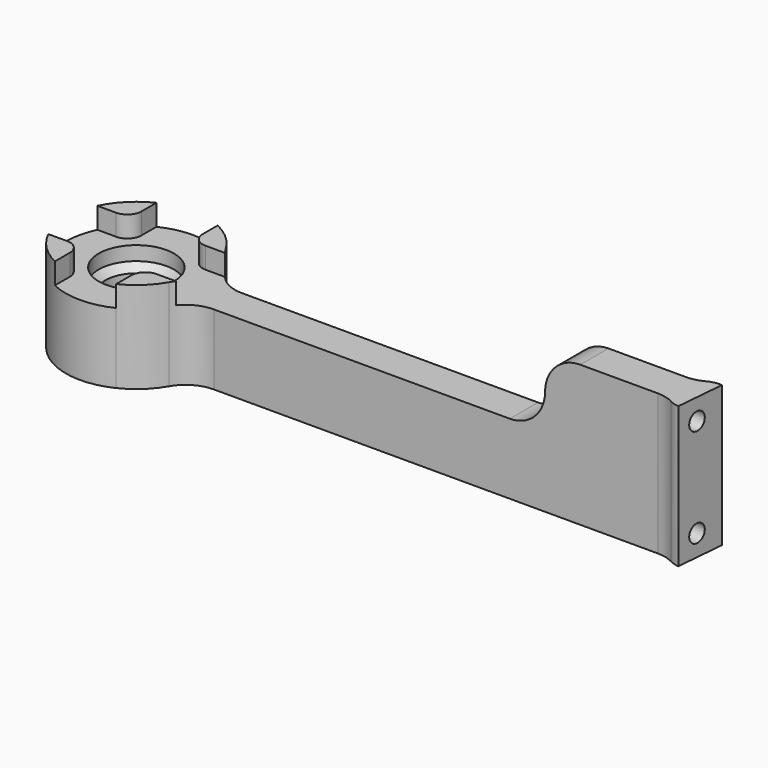
from build123d import *

# Parameters (mm, degrees)
F0_R         = 5.35
F1_DEPTH     = 10
F2_START     = 3.5
F0_R_2       = 4.35
F2_DEPTH     = 4.5
F3_SIZE      = 0.99999
F4_DEPTH     = 13
F5_DEPTH     = 20
F6_R         = 1.25
F7_DEPTH     = 7.5
F8_T1_DEPTH  = 20
F8_T3_DEPTH  = 5
F8_T8_DEPTH  = 10
F8_T13_DEPTH = 10
F8_T18_DEPTH = 18.2698067281
F8_T25_DEPTH = 10
F8_T30_DEPTH = 10
F8_T35_DEPTH = 18.2698067281
F8_T39_DEPTH = 30


# Not quite as in the source:
# - a fillet or chamfer that OpenCascade refuses, or shapes differently, is made with other operations: its cross-section is extruded or revolved along the edge and cut away or added
# - a fillet or chamfer is up to 0.001 mm smaller than in the source, because OpenCascade refuses the exact size


with BuildPart() as f1:
    # F0 (on Top) → F1 (new body)
    with BuildSketch(Plane.XY):
        with BuildLine():
            Line((-4.35, 6.35), (-4.35, 9.0043045262))
            ThreePointArc((-4.35, 9.0043045262), (-7.0710678119, 7.0710678119), (-9.0043045262, 4.35))
            Line((-9.0043045262, 4.35), (-6.35, 4.35))
            ThreePointArc((-6.35, 4.35), (-4.9357864376, 4.9357864376), (-4.35, 6.35))
        make_face()
        with BuildLine():
            ThreePointArc((9.6824583655, -2.5), (9.9202969627, -1.2600429248), (10, 0))
            ThreePointArc((10, 0), (9.9202969627, 1.2600429248), (9.6824583655, 2.5))
            ThreePointArc((9.6824583655, 2.5), (9.3890575588, 3.4417434764), (9.0043045262, 4.35))
            Line((9.0043045262, 4.35), (6.35, 4.35))
            ThreePointArc((6.35, 4.35), (4.9357864376, 4.9357864376), (4.35, 6.35))
            Line((4.35, 6.35), (4.35, 9.0043045262))
            ThreePointArc((4.35, 9.0043045262), (0, 10), (-4.35, 9.0043045262))
            Line((-4.35, 9.0043045262), (-4.35, 6.35))
            ThreePointArc((-4.35, 6.35), (-4.9357864376, 4.9357864376), (-6.35, 4.35))
            Line((-6.35, 4.35), (-9.0043045262, 4.35))
            ThreePointArc((-9.0043045262, 4.35), (-10, 0), (-9.0043045262, -4.35))
            Line((-9.0043045262, -4.35), (-6.35, -4.35))
            ThreePointArc((-6.35, -4.35), (-4.9357864376, -4.9357864376), (-4.35, -6.35))
            Line((-4.35, -6.35), (-4.35, -9.0043045262))
            ThreePointArc((-4.35, -9.0043045262), (0, -10), (4.35, -9.0043045262))
            Line((4.35, -9.0043045262), (4.35, -6.35))
            ThreePointArc((4.35, -6.35), (4.9357864376, -4.9357864376), (6.35, -4.35))
            Line((6.35, -4.35), (9.0043045262, -4.35))
            ThreePointArc((9.0043045262, -4.35), (9.3890575588, -3.4417434764), (9.6824583655, -2.5))
        make_face()
        Circle(F0_R, mode=Mode.SUBTRACT)
        with BuildLine():
            ThreePointArc((-9.0043045262, -4.35), (-7.0710678119, -7.0710678119), (-4.35, -9.0043045262))
            Line((-4.35, -9.0043045262), (-4.35, -6.35))
            ThreePointArc((-4.35, -6.35), (-4.9357864376, -4.9357864376), (-6.35, -4.35))
            Line((-6.35, -4.35), (-9.0043045262, -4.35))
        make_face()
        with BuildLine():
            ThreePointArc((4.35, -9.0043045262), (7.0710678119, -7.0710678119), (9.0043045262, -4.35))
            Line((9.0043045262, -4.35), (6.35, -4.35))
            ThreePointArc((6.35, -4.35), (4.9357864376, -4.9357864376), (4.35, -6.35))
            Line((4.35, -6.35), (4.35, -9.0043045262))
        make_face()
        with BuildLine():
            Line((6.35, 4.35), (9.0043045262, 4.35))
            ThreePointArc((9.0043045262, 4.35), (7.0710678119, 7.0710678119), (4.35, 9.0043045262))
            Line((4.35, 9.0043045262), (4.35, 6.35))
            ThreePointArc((4.35, 6.35), (4.9357864376, 4.9357864376), (6.35, 4.35))
        make_face()
        with BuildLine():
            ThreePointArc((9.6824583655, 2.5), (9.9202969627, 1.2600429248), (10, 0))
            ThreePointArc((10, 0), (9.9202969627, -1.2600429248), (9.6824583655, -2.5))
            Line((9.6824583655, -2.5), (60, -2.5))
            Line((60, -2.5), (60, 2.5))
            Line((60, 2.5), (9.6824583655, 2.5))
        make_face()
        with BuildLine():
            Line((77.5505102572, 2.5), (60, 2.5))
            Line((60, 2.5), (60, -2.5))
            Line((60, -2.5), (77.5505102572, -2.5))
            ThreePointArc((77.5505102572, -2.5), (76.5, 0), (77.5505102572, 2.5))
        make_face()
        with BuildLine():
            ThreePointArc((80.3050450996, 3.4866814433), (78.8197263984, 3.2949892603), (77.5505102572, 2.5))
            ThreePointArc((77.5505102572, 2.5), (76.5, 0), (77.5505102572, -2.5))
            ThreePointArc((77.5505102572, -2.5), (78.5370404595, -3.179583209), (79.6949549004, -3.4866814433))
            Line((79.6949549004, -3.4866814433), (80, 0))
            Line((80, 0), (80.3050450996, 3.4866814433))
        make_face()
    extrude(amount=F1_DEPTH)

    # F0 (on Top) → F2 (join)
    with BuildSketch(Plane.XY.offset(F2_START)):
        Circle(F0_R)
        Circle(F0_R_2, mode=Mode.SUBTRACT)
    extrude(amount=F2_DEPTH)

    # F3 (size 1 in the source; OpenCascade refuses exactly that, so slightly less here)
    f3_edges = [f1.edges().sort_by_distance(p)[0] for p in [
        (-4.35, 0, 3.5),
        (-4.35, 0, 8),
    ]]
    chamfer(f3_edges, length=F3_SIZE)

    # F0 (on Top) → F4 (join)
    with BuildSketch(Plane.XY):
        with BuildLine():
            ThreePointArc((-9.0043045262, -4.35), (-7.0710678119, -7.0710678119), (-4.35, -9.0043045262))
            Line((-4.35, -9.0043045262), (-4.35, -6.35))
            ThreePointArc((-4.35, -6.35), (-4.9357864376, -4.9357864376), (-6.35, -4.35))
            Line((-6.35, -4.35), (-9.0043045262, -4.35))
        make_face()
        with BuildLine():
            ThreePointArc((4.35, -9.0043045262), (7.0710678119, -7.0710678119), (9.0043045262, -4.35))
            Line((9.0043045262, -4.35), (6.35, -4.35))
            ThreePointArc((6.35, -4.35), (4.9357864376, -4.9357864376), (4.35, -6.35))
            Line((4.35, -6.35), (4.35, -9.0043045262))
        make_face()
        with BuildLine():
            Line((6.35, 4.35), (9.0043045262, 4.35))
            ThreePointArc((9.0043045262, 4.35), (7.0710678119, 7.0710678119), (4.35, 9.0043045262))
            Line((4.35, 9.0043045262), (4.35, 6.35))
            ThreePointArc((4.35, 6.35), (4.9357864376, 4.9357864376), (6.35, 4.35))
        make_face()
        with BuildLine():
            Line((-4.35, 6.35), (-4.35, 9.0043045262))
            ThreePointArc((-4.35, 9.0043045262), (-7.0710678119, 7.0710678119), (-9.0043045262, 4.35))
            Line((-9.0043045262, 4.35), (-6.35, 4.35))
            ThreePointArc((-6.35, 4.35), (-4.9357864376, 4.9357864376), (-4.35, 6.35))
        make_face()
    extrude(amount=F4_DEPTH)

    # F0 (on Top) → F5 (join)
    with BuildSketch(Plane.XY):
        with BuildLine():
            ThreePointArc((80.3050450996, 3.4866814433), (78.8197263984, 3.2949892603), (77.5505102572, 2.5))
            ThreePointArc((77.5505102572, 2.5), (76.5, 0), (77.5505102572, -2.5))
            ThreePointArc((77.5505102572, -2.5), (78.5370404595, -3.179583209), (79.6949549004, -3.4866814433))
            Line((79.6949549004, -3.4866814433), (80, 0))
            Line((80, 0), (80.3050450996, 3.4866814433))
        make_face()
        with BuildLine():
            Line((77.5505102572, 2.5), (60, 2.5))
            Line((60, 2.5), (60, -2.5))
            Line((60, -2.5), (77.5505102572, -2.5))
            ThreePointArc((77.5505102572, -2.5), (76.5, 0), (77.5505102572, 2.5))
        make_face()
    extrude(amount=F5_DEPTH)

    # F6 (on face) → F7 (cut)
    with BuildSketch(Plane(origin=(79.3923101205, -6.9459271067, 0), x_dir=(0.0871557427, 0.9961946981, 0), z_dir=(0.9961946981, -0.0871557427, 0))):
        with Locations((6.4724594198, 17)):
            Circle(F6_R)
        with Locations((6.4724594198, 3)):
            Circle(F6_R)
    extrude(amount=-F7_DEPTH, mode=Mode.SUBTRACT)

    # F8: fillet of radius 5 on 6 edges, made by hand

    # F8_s2 → F8_t1 (join)
    with BuildSketch(Plane.XY):
        with BuildLine():
            ThreePointArc((78.3529411765, 3.0882352941), (77.2126781252, 2.6492874993), (76, 2.5))
            Line((76, 2.5), (77.5505102572, 2.5))
            ThreePointArc((77.5505102572, 2.5), (77.9307168562, 2.822776518), (78.3529411765, 3.0882352941))
        make_face()
        with BuildLine():
            ThreePointArc((76, -2.5), (77.2126781252, -2.6492874993), (78.3529411765, -3.0882352941))
            ThreePointArc((78.3529411765, -3.0882352941), (77.9307168562, -2.822776518), (77.5505102572, -2.5))
            Line((77.5505102572, -2.5), (76, -2.5))
        make_face()
    extrude(amount=F8_T1_DEPTH)

    # F8_s4 → F8_t3 (join)
    with BuildSketch(Plane.XZ.offset(-2.5)):
        with BuildLine():
            ThreePointArc((55, 10), (58.5355339059, 11.4644660941), (60, 15))
            Line((60, 15), (60, 10))
            Line((60, 10), (55, 10))
        make_face()
    extrude(amount=F8_T3_DEPTH)


with BuildPart() as f8_tool6:
    # F8_s7 → F8_t8 (new body)
    with BuildSketch(Plane.XY):
        with BuildLine():
            ThreePointArc((8.6602540378, 5), (10.4903810568, 3.1698729811), (12.9903810568, 2.5))
            Line((12.9903810568, 2.5), (9.6824583655, 2.5))
            ThreePointArc((9.6824583655, 2.5), (9.2561479341, 3.7846697903), (8.6602540378, 5))
        make_face()
    extrude(amount=F8_T8_DEPTH)

    split(bisect_by=Plane.XZ.offset(-4.35), keep=Keep.BOTTOM)


with BuildPart() as f1_1:
    add(f1.part)

    # F8_t5: union F8_tool6
    add(f8_tool6.part)


with BuildPart() as f8_tool11:
    # F8_s12 → F8_t13 (new body)
    with BuildSketch(Plane.XY):
        with BuildLine():
            ThreePointArc((8.6602540378, 5), (10.4903810568, 3.1698729811), (12.9903810568, 2.5))
            Line((12.9903810568, 2.5), (9.6824583655, 2.5))
            ThreePointArc((9.6824583655, 2.5), (9.2561479341, 3.7846697903), (8.6602540378, 5))
        make_face()
    extrude(amount=F8_T13_DEPTH)

    split(bisect_by=Plane.XZ.offset(-4.35), keep=Keep.TOP)


with BuildPart() as f1_2:
    add(f1_1.part)

    # F8_t10: union F8_tool11
    add(f8_tool11.part)


with BuildPart() as f8_tool16:
    # F8_s17 → F8_t18 (new body)
    with BuildSketch(Plane.XY):
        with BuildLine():
            ThreePointArc((8.6602540378, 5), (10.4903810568, 3.1698729811), (12.9903810568, 2.5))
            Line((12.9903810568, 2.5), (9.6824583655, 2.5))
            ThreePointArc((9.6824583655, 2.5), (9.2561479341, 3.7846697903), (8.6602540378, 5))
        make_face()
    extrude(amount=F8_T18_DEPTH)

    split(bisect_by=Plane.XY.offset(10), keep=Keep.TOP)

    split(bisect_by=Plane.XZ.offset(-4.35), keep=Keep.BOTTOM)

    split(bisect_by=Plane.XY.offset(13), keep=Keep.BOTTOM)


with BuildPart() as f1_3:
    add(f1_2.part)

    # F8_t15: union F8_tool16
    add(f8_tool16.part)


with BuildPart() as f8_tool23:
    # F8_s24 → F8_t25 (new body)
    with BuildSketch(Plane.XY):
        with BuildLine():
            ThreePointArc((8.6602540378, -5), (10.4903810568, -3.1698729811), (12.9903810568, -2.5))
            Line((12.9903810568, -2.5), (9.6824583655, -2.5))
            ThreePointArc((9.6824583655, -2.5), (9.2561479341, -3.7846697903), (8.6602540378, -5))
        make_face()
    extrude(amount=F8_T25_DEPTH)

    split(bisect_by=Plane.XZ.offset(4.35), keep=Keep.TOP)


with BuildPart() as f1_4:
    add(f1_3.part)

    # F8_t22: union F8_tool23
    add(f8_tool23.part)


with BuildPart() as f8_tool28:
    # F8_s29 → F8_t30 (new body)
    with BuildSketch(Plane.XY):
        with BuildLine():
            ThreePointArc((8.6602540378, -5), (10.4903810568, -3.1698729811), (12.9903810568, -2.5))
            Line((12.9903810568, -2.5), (9.6824583655, -2.5))
            ThreePointArc((9.6824583655, -2.5), (9.2561479341, -3.7846697903), (8.6602540378, -5))
        make_face()
    extrude(amount=F8_T30_DEPTH)

    split(bisect_by=Plane.XZ.offset(4.35), keep=Keep.BOTTOM)


with BuildPart() as f1_5:
    add(f1_4.part)

    # F8_t27: union F8_tool28
    add(f8_tool28.part)


with BuildPart() as f8_tool33:
    # F8_s34 → F8_t35 (new body)
    with BuildSketch(Plane.XY):
        with BuildLine():
            ThreePointArc((8.6602540378, -5), (10.4903810568, -3.1698729811), (12.9903810568, -2.5))
            Line((12.9903810568, -2.5), (9.6824583655, -2.5))
            ThreePointArc((9.6824583655, -2.5), (9.2561479341, -3.7846697903), (8.6602540378, -5))
        make_face()
    extrude(amount=F8_T35_DEPTH)

    split(bisect_by=Plane.XY.offset(10), keep=Keep.TOP)

    split(bisect_by=Plane.XY.offset(13), keep=Keep.BOTTOM)

    split(bisect_by=Plane.XZ.offset(4.35), keep=Keep.TOP)


with BuildPart() as f1_6:
    add(f1_5.part)

    # F8_t32: union F8_tool33
    add(f8_tool33.part)

    # F8_s40 → F8_t39 (cut)
    with BuildSketch(Plane.XZ.offset(-15)):
        with BuildLine():
            ThreePointArc((60, 15), (61.4644660941, 18.5355339059), (65, 20))
            Line((65, 20), (60, 20))
            Line((60, 20), (60, 15))
        make_face()
    extrude(amount=F8_T39_DEPTH, mode=Mode.SUBTRACT)


solid = f1_6.part
